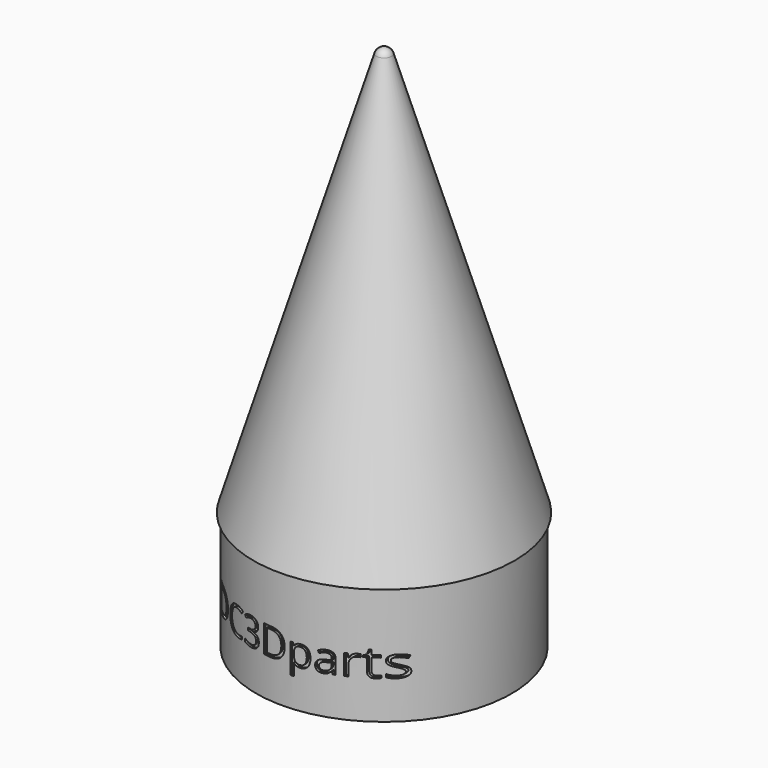
from build123d import *

# Parameters (mm, degrees)
F3_TEXT_SIZE = 9.7222222222
F4_DEPTH     = 40
F5_W         = 32
F5_H         = 30.6678369078


# Not quite as in the source:
# - Text() gives the source's letters only with a copy of the font that has no kerning and outlines rounded to 1/6400 em; it was checked with that copy


with BuildPart() as f1:
    # F0 (on Front) → F1 (revolve)
    with BuildSketch(Plane.XZ):
        with BuildLine():
            Line((-32.55, -30), (0, -30))
            Line((0, -30), (0, 0))
            Line((0, 0), (0, 78.7014423827))
            Line((0, 78.7014423827), (0, 104.2418664922))
            ThreePointArc((0, 104.2418664922), (-1.1937062605, 103.8479350801), (-1.9184808616, 102.82089157))
            Line((-1.9184808616, 102.82089157), (-33.25, 0))
            Line((-33.25, 0), (-32.55, 0))
            Line((-32.55, 0), (-32.55, -30))
        make_face()
    revolve(axis=Axis((0, 0, 1.4177560806), (0, 0, -1)))


with BuildPart() as f4:
    # F3 (on offset) → F4 (new body, through all)
    with BuildSketch(Plane.XZ.offset(40)):
        with Locations((-24.5241850537, -20.2161904941)):
            Text('DC3Dparts', F3_TEXT_SIZE, font='Open Sans', text_align=(TextAlign.LEFT, TextAlign.BOTTOM))
    extrude(amount=-F4_DEPTH)


with BuildPart() as f6:
    # F5 (on Front) → F6 (revolve)
    with BuildSketch(Plane.XZ):
        with Locations((-16, -18.3048572447)):
            Rectangle(F5_W, F5_H)
    revolve(axis=Axis((0, 0, -18.3048572447), (0, 0, -1)))


with BuildPart() as f4_1:
    add(f4.part)

    # F7: cut F6
    add(f6.part, mode=Mode.SUBTRACT)


with BuildPart() as f1_1:
    add(f1.part)

    # F8: cut F4
    add(f4_1.part, mode=Mode.SUBTRACT)


solid = f1_1.part
